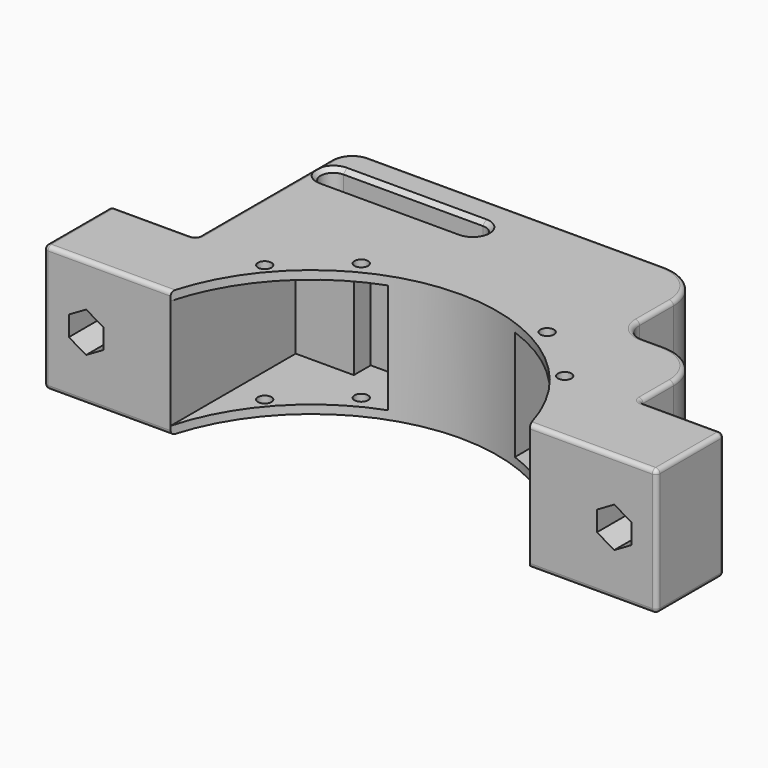
from build123d import *

# Parameters (mm, degrees)
F1_DEPTH       = 30
F3_W           = 27.5
F3_H           = 26
F4_DEPTH       = 37
F7_DEPTH       = 20.001
F9_W           = 13.75
F9_H           = 26
F10_W          = 13.75
F10_H          = 26
F11_DEPTH      = 5
F8_R           = 1.6
F12_DEPTH      = 2.001
F12_DEPTH_BACK = 28.001
F13_W          = 32.5
F13_H          = 20
F14_DEPTH      = 20
F15_DEPTH      = 20
F17_DEPTH      = 10.001
F18_R          = 10
F19_R          = 5
F20_R          = 1
F21_T1_DEPTH   = 33
F21_T4_ANGLE   = 180
F21_T6_ANGLE   = 180
F21_T8_ANGLE   = 180
F21_T10_ANGLE  = 180


# Not quite as in the source:
# - a fillet or chamfer that OpenCascade refuses, or shapes differently, is made with other operations: its cross-section is extruded or revolved along the edge and cut away or added


with BuildPart() as f1:
    # F0 (on Top) → F1 (new body)
    with BuildSketch(Plane.XY):
        with BuildLine():
            Line((-52.7744764373, 20.2577475536), (-52.7744764373, 0.2577475536))
            Line((-52.7744764373, 0.2577475536), (-22.7744764373, 0.2577475536))
            ThreePointArc((-22.7744764373, 0.2577475536), (19.7255235627, 32.8669618037), (62.2255235627, 0.2577475536))
            Line((62.2255235627, 0.2577475536), (92.2255235627, 0.2577475536))
            Line((92.2255235627, 0.2577475536), (92.2255235627, 20.2577475536))
            Line((92.2255235627, 20.2577475536), (72.2255235627, 20.2577475536))
            Line((72.2255235627, 20.2577475536), (72.2255235627, 40.2577475536))
            Line((72.2255235627, 40.2577475536), (52.2255235627, 40.2577475536))
            Line((52.2255235627, 40.2577475536), (52.2255235627, 65.2577475536))
            Line((52.2255235627, 65.2577475536), (-12.7744764373, 65.2577475536))
            Line((-12.7744764373, 65.2577475536), (-12.7744764373, 40.2577475536))
            Line((-12.7744764373, 40.2577475536), (-32.7744764373, 40.2577475536))
            Line((-32.7744764373, 40.2577475536), (-32.7744764373, 20.2577475536))
            Line((-32.7744764373, 20.2577475536), (-52.7744764373, 20.2577475536))
        make_face()
    extrude(amount=F1_DEPTH)

    # F3 (on offset) → F4 (cut)
    with BuildSketch(Plane.XZ.offset(-0.2577475536)):
        with Locations((-9.0244764373, 15)):
            Rectangle(F3_W, F3_H)
        with Locations((48.4755235627, 15)):
            Rectangle(F3_W, F3_H)
    extrude(amount=-F4_DEPTH, mode=Mode.SUBTRACT)

    # F6 (on face) + F5 (on face) → F7 (cut, through all)
    with BuildSketch(Plane(origin=(0, 20.2577475536, 0), x_dir=(-1, 0, 0), z_dir=(0, 1, 0))):
        Polygon((-86.3255235627, 17.3671361037), (-86.3255235627, 12.6328638963), (-82.2255235627, 10.2657277926), (-78.1255235627, 12.6328638963), (-78.1255235627, 17.3671361037), (-82.2255235627, 19.7342722074), align=None)
    with BuildSketch(Plane(origin=(0, 20.2577475536, 0), x_dir=(-1, 0, 0), z_dir=(0, 1, 0))):
        Polygon((42.7744764373, 10.2657277926), (46.8744764373, 12.6328638963), (46.8744764373, 17.3671361037), (42.7744764373, 19.7342722074), (38.6744764373, 17.3671361037), (38.6744764373, 12.6328638963), align=None)
    extrude(amount=-F7_DEPTH, mode=Mode.SUBTRACT)

    # F9 (on face) + F10 (on face) → F11 (cut)
    with BuildSketch(Plane.XZ.offset(-37.2577475536)):
        with Locations((41.6005235627, 15)):
            Rectangle(F9_W, F9_H)
    with BuildSketch(Plane.XZ.offset(-37.2577475536)):
        with Locations((-2.1494764373, 15)):
            Rectangle(F10_W, F10_H)
    extrude(amount=-F11_DEPTH, mode=Mode.SUBTRACT)

    # F8 (on face) → F12 (cut, two sides)
    with BuildSketch(Plane(origin=(0, 0, 28), x_dir=(1, 0, 0), z_dir=(0, 0, -1))) as f12_sk:
        with Locations((55.2255235627, -19.3357891615)):
            Circle(F8_R)
        with Locations((41.7255235627, -31.033055583)):
            Circle(F8_R)
        with Locations((-15.7744764373, -19.3357891615)):
            Circle(F8_R)
        with Locations((-2.2744764373, -31.033055583)):
            Circle(F8_R)
    extrude(amount=-F12_DEPTH, mode=Mode.SUBTRACT)
    extrude(f12_sk.sketch, amount=F12_DEPTH_BACK, mode=Mode.SUBTRACT)

    # F13 (on face) → F14 (cut)
    with BuildSketch(Plane(origin=(0, 0, 0), x_dir=(1, 0, 0), z_dir=(0, 0, -1))):
        with Locations((3.4755235627, -55.2577475536)):
            Rectangle(F13_W, F13_H)
    extrude(amount=-F14_DEPTH, mode=Mode.SUBTRACT)

    # F15 (add, through all): a face of the model
    f15_faces = [f1.faces().sort_by_distance(p)[0] for p in [
        (-12.7744764373, 49.9006046965, 20.7142857143),
    ]]
    extrude(f15_faces, amount=F15_DEPTH)

    # F16 (on face) → F17 (cut, through all)
    with BuildSketch(Plane(origin=(0, 0, 20), x_dir=(1, 0, 0), z_dir=(0, 0, -1))):
        with BuildLine():
            Line((-28.2744764373, -58.2577475536), (4.7255235627, -58.2577475536))
            ThreePointArc((4.7255235627, -58.2577475536), (7.7255235627, -55.2577475536), (4.7255235627, -52.2577475536))
            Line((4.7255235627, -52.2577475536), (-28.2744764373, -52.2577475536))
            ThreePointArc((-28.2744764373, -52.2577475536), (-31.2744764373, -55.2577475536), (-28.2744764373, -58.2577475536))
        make_face()
    extrude(amount=-F17_DEPTH, mode=Mode.SUBTRACT)

    # F18
    f18_edges = [f1.edges().sort_by_distance(p)[0] for p in [
        (52.225524, 65.257748, 15),
        (72.225524, 40.257748, 15),
    ]]
    fillet(f18_edges, radius=F18_R)

    # F19
    f19_edges = [f1.edges().sort_by_distance(p)[0] for p in [
        (52.225524, 40.257748, 15),
        (-32.774476, 65.257748, 25),
        (-32.774476, 45.257748, 10),
    ]]
    fillet(f19_edges, radius=F19_R)

    # F20
    f20_edges = [f1.edges().sort_by_distance(p)[0] for p in [
        (82.225524, 20.257748, 30),
        (92.225524, 10.257748, 30),
        (77.225524, 0.257748, 30),
        (92.225524, 0.257748, 15),
        (77.225524, 0.257748, 0),
        (92.225524, 10.257748, 0),
        (82.225524, 20.257748, 0),
        (92.225524, 20.257748, 15),
        (72.225524, 20.257748, 15),
        (-42.774476, 20.257748, 30),
        (-37.774476, 0.257748, 30),
        (-52.774476, 10.257748, 30),
        (-52.774476, 20.257748, 15),
        (-52.774476, 0.257748, 15),
        (-37.774476, 0.257748, 0),
        (-52.774476, 10.257748, 0),
        (-42.774476, 20.257748, 0),
        (-32.774476, 20.257748, 15),
        (19.725524, 55.257748, 0),
        (19.725524, 65.257748, 10),
        (-4.024476, 65.257748, 20),
        (59.725524, 40.257748, 0),
        (53.68999, 41.722214, 0),
        (69.296591, 37.328815, 0),
        (52.225524, 50.257748, 0),
        (72.225524, 25.257748, 0),
        (49.296591, 62.328815, 0),
        (30.975524, 65.257748, 0),
        (-4.024476, 45.257748, 0),
        (-31.31001, 43.793281, 0),
        (-32.774476, 30.257748, 0),
        (59.725524, 40.257748, 30),
        (53.68999, 41.722214, 30),
        (69.296591, 37.328815, 30),
        (52.225524, 50.257748, 30),
        (72.225524, 25.257748, 30),
        (49.296591, 62.328815, 30),
        (7.225524, 65.257748, 30),
        (-32.774476, 42.757748, 20),
        (-32.774476, 40.257748, 30),
        (-32.774476, 52.757748, 20),
        (-31.31001, 63.793281, 30),
        (-31.31001, 63.793281, 20),
    ]]
    fillet(f20_edges, radius=F20_R)

    # F21: chamfer of 1 on 8 edges, made by hand

    # F21_s2 → F21_t1 (cut)
    with BuildSketch(Plane.YZ.offset(-28.2744764373)):
        Polygon((58.2577475536, 21), (59.2577475536, 20), (58.2577475536, 20), align=None)
        Polygon((52.2577475536, 21), (51.2577475536, 20), (52.2577475536, 20), align=None)
        Polygon((59.2577475536, 30), (58.2577475536, 29), (58.2577475536, 30), align=None)
        Polygon((51.2577475536, 30), (52.2577475536, 29), (52.2577475536, 30), align=None)
    extrude(amount=F21_T1_DEPTH, mode=Mode.SUBTRACT)

    # F21_s3 → F21_t4 (revolve, cut)
    with BuildSketch(Plane.YZ.offset(4.7255235627)):
        Polygon((58.2577475536, 21), (59.2577475536, 20), (58.2577475536, 20), align=None)
    revolve(axis=Axis((4.7255235627, 55.2577475536, 20), (0, 0, -1)), revolution_arc=F21_T4_ANGLE, mode=Mode.SUBTRACT)

    # F21_s5 → F21_t6 (revolve, cut)
    with BuildSketch(Plane.YZ.offset(-28.2744764373)):
        Polygon((52.2577475536, 21), (51.2577475536, 20), (52.2577475536, 20), align=None)
    revolve(axis=Axis((-28.2744764373, 55.2577475536, 20), (0, 0, -1)), revolution_arc=F21_T6_ANGLE, mode=Mode.SUBTRACT)

    # F21_s7 → F21_t8 (revolve, cut)
    with BuildSketch(Plane.YZ.offset(-28.2744764373)):
        Polygon((51.2577475536, 30), (52.2577475536, 29), (52.2577475536, 30), align=None)
    revolve(axis=Axis((-28.2744764373, 55.2577475536, 30), (0, 0, -1)), revolution_arc=F21_T8_ANGLE, mode=Mode.SUBTRACT)

    # F21_s9 → F21_t10 (revolve, cut)
    with BuildSketch(Plane.YZ.offset(4.7255235627)):
        Polygon((59.2577475536, 30), (58.2577475536, 29), (58.2577475536, 30), align=None)
    revolve(axis=Axis((4.7255235627, 55.2577475536, 30), (0, 0, -1)), revolution_arc=F21_T10_ANGLE, mode=Mode.SUBTRACT)


solid = f1.part
